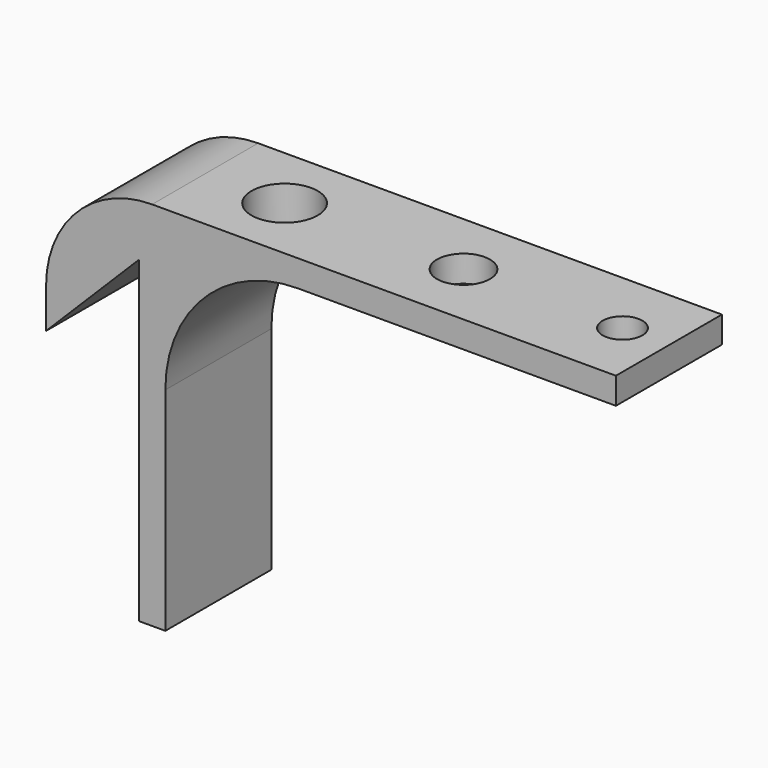
from build123d import *

# Parameters (mm, degrees)
F1_DEPTH = 25.4
F2_R     = 3.81
F2_R_2   = 5.08
F2_R_3   = 6.35
F3_DEPTH = 71.1383146132


# Not quite as in the source:
# - a feature names something its author has since deleted; it is built from what else it names


with BuildPart() as f1:
    # F0 (on Front) → F1 (new body)
    with BuildSketch(Plane.XZ):
        with BuildLine():
            Line((-5.08, 0), (0, 0))
            Line((0, 0), (0, 38.1))
            Line((0, 38.1), (0, 40.6573146132))
            ThreePointArc((0, 40.6573146132), (7.4394877579, 58.6178268553), (25.4, 66.0573146132))
            Line((25.4, 66.0573146132), (86.36, 66.0573146132))
            Line((86.36, 66.0573146132), (86.36, 71.1373146132))
            Line((86.36, 71.1373146132), (0, 71.1373146132))
            Line((0, 71.1373146132), (-2.54, 71.1373146132))
            ThreePointArc((-2.54, 71.1373146132), (-16.9084097937, 65.1857244069), (-22.86, 50.8173146132))
            Line((-22.86, 50.8173146132), (-22.86, 43.18))
            Line((-22.86, 43.18), (-5.08, 60.96))
            Line((-5.08, 60.96), (-5.08, 0))
        make_face()
    extrude(amount=F1_DEPTH)

    # F2 (on face) → F3 (cut, through all)
    with BuildSketch(Plane.XY.offset(71.1373146132)):
        with Locations((77.47, -12.7)):
            Circle(F2_R)
        with Locations((46.99, -12.7)):
            Circle(F2_R_2)
        with Locations((12.7, -12.7)):
            Circle(F2_R_3)
    extrude(amount=-F3_DEPTH, mode=Mode.SUBTRACT)


solid = f1.part
